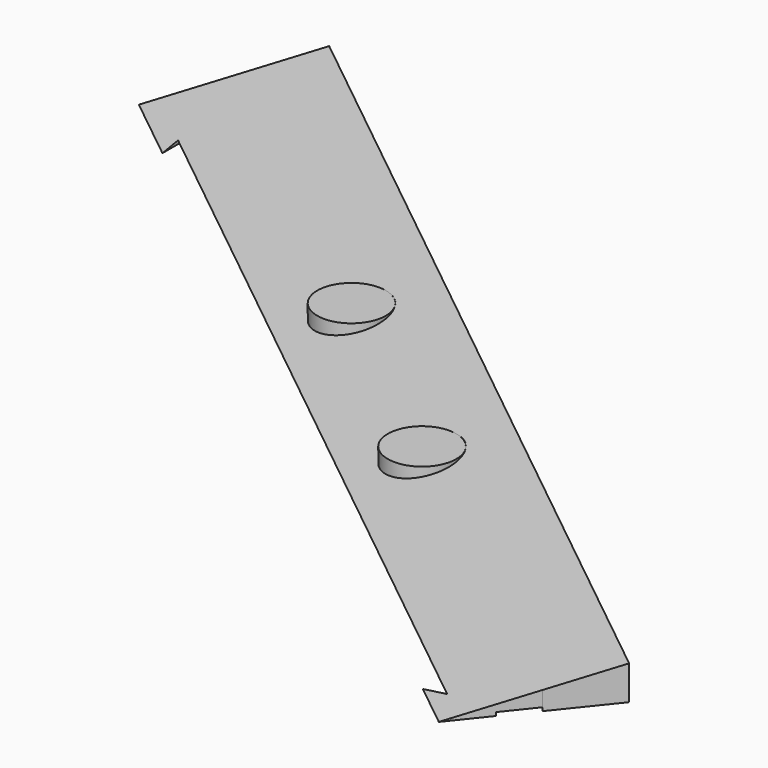
from build123d import *
from build123d import SkipClean  # not in build123d's __all__

# Parameters (mm, degrees)
F0_R     = 10
F1_DEPTH = 10
F2_DEPTH = 1
F4_DEPTH = 345
F5_DEPTH = 7.3
F6_DEPTH = 1.6


with BuildPart() as f1:
    # F0 (on Top) → F1 (new body)
    with BuildSketch(Plane.XY):
        Polygon((-255.5560874402, 235.83927431), (-264.2086340252, 225.0363213116), (-264.2086340252, 185.7455475346), (-236.384913462, 220.4842620314), align=None)
        Polygon((-264.2086340252, 185.7455475346), (-264.2086340252, 225.0363213116), (-283.3798080034, 201.1005598132), align=None)
        Polygon((-236.384913462, 220.4842620314), (-264.2086340252, 185.7455475346), (-236.8907927142, 163.8655213438), (-209.0670721511, 198.6042358405), align=None)
        Polygon((-209.0670721511, 198.6042358405), (-236.8907927142, 163.8655213438), (-108.6030207612, 61.1143640196), (-80.779300198, 95.8530785163), align=None)
        with Locations((-175.4610245732, 143.8843668861)):
            Circle(F0_R, mode=Mode.SUBTRACT)
        with Locations((-118.6635494232, 98.6492335796)):
            Circle(F0_R, mode=Mode.SUBTRACT)
        Polygon((-80.779300198, 95.8530785163), (-108.6030207612, 61.1143640196), (-52.4192279143, 16.1143640196), (-31.023575784, 16.1143640196), (-24.2086340252, 24.6230145983), (-24.2086340252, 50.5432151414), align=None)
        Polygon((-11.5613729408, 40.4134834171), (-24.2086340252, 50.5432151414), (-24.2086340252, 24.6230145983), align=None)
        Polygon((-31.023575784, 16.1143640196), (-52.4192279143, 16.1143640196), (-39.385093504, 5.6747689203), align=None)
    extrude(amount=F1_DEPTH)

    # F0 (on Top) → F2 (cut)
    with BuildSketch(Plane.XY):
        Polygon((-255.5560874402, 235.83927431), (-264.2086340252, 225.0363213116), (-264.2086340252, 185.7455475346), (-236.384913462, 220.4842620314), align=None)
        Polygon((-236.384913462, 220.4842620314), (-264.2086340252, 185.7455475346), (-236.8907927142, 163.8655213438), (-209.0670721511, 198.6042358405), align=None)
        Polygon((-209.0670721511, 198.6042358405), (-236.8907927142, 163.8655213438), (-108.6030207612, 61.1143640196), (-80.779300198, 95.8530785163), align=None)
        with Locations((-175.4610245732, 143.8843668861)):
            Circle(F0_R, mode=Mode.SUBTRACT)
        with Locations((-118.6635494232, 98.6492335796)):
            Circle(F0_R, mode=Mode.SUBTRACT)
        Polygon((-80.779300198, 95.8530785163), (-108.6030207612, 61.1143640196), (-52.4192279143, 16.1143640196), (-31.023575784, 16.1143640196), (-24.2086340252, 24.6230145983), (-24.2086340252, 50.5432151414), align=None)
    extrude(amount=F2_DEPTH, mode=Mode.SUBTRACT)

    # F3 (on face) → F4 (cut)
    with BuildSketch(Plane(origin=(-270.7568290083, 216.860711746, 0), x_dir=(-0.6251436055, -0.7805097517, 0), z_dir=(-0.7805097517, 0.6251436055, 0))):
        Polygon((20.192126873, 10), (-24.3155995446, 10), (20.192126873, 0), align=None)
        Polygon((-17.6889132261, 39.4938741719), (-24.3155995446, 10), (20.192126873, 10), (20.192126873, 0), (26.8188131915, 29.4938741719), align=None)
    extrude(amount=-F4_DEPTH, mode=Mode.SUBTRACT)

    # F0 (on Top) → F5 (join)
    with BuildSketch(Plane.XY):
        with Locations((-175.4610245732, 143.8843668861)):
            Circle(F0_R)
        with Locations((-118.6635494232, 98.6492335796)):
            Circle(F0_R)
    with SkipClean():  # cleaning this boolean's faces spoils the solid; the shape is the same uncleaned
        extrude(amount=F5_DEPTH)

    # F0 (on Top) → F6 (cut)
    with BuildSketch(Plane.XY):
        with Locations((-118.6635494232, 98.6492335796)):
            Circle(F0_R)
        with Locations((-175.4610245732, 143.8843668861)):
            Circle(F0_R)
    with SkipClean():  # cleaning this boolean's faces spoils the solid; the shape is the same uncleaned
        extrude(amount=F6_DEPTH, mode=Mode.SUBTRACT)


solid = f1.part
